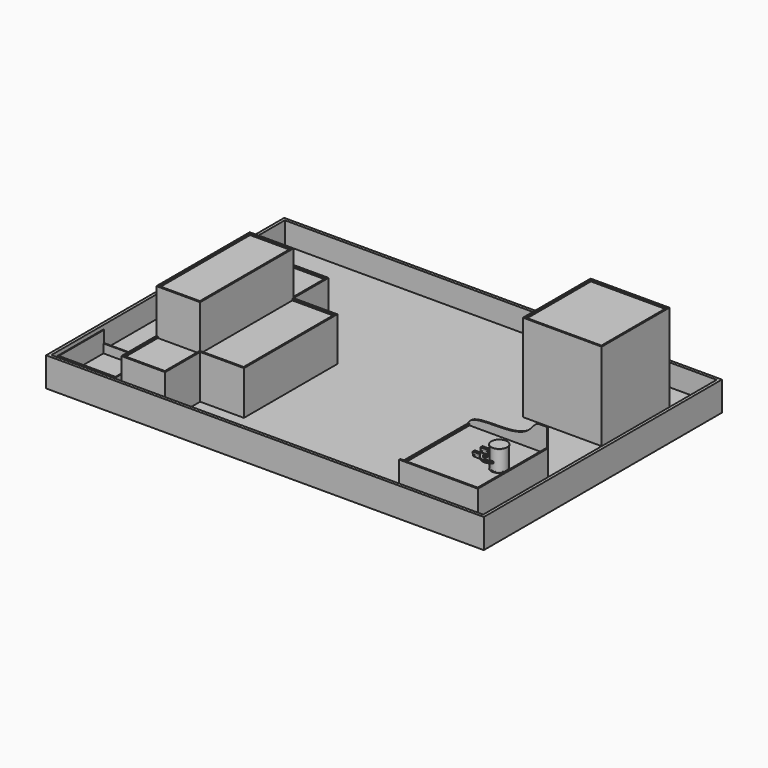
from build123d import *

# Parameters (mm, degrees)
F0_R      = 27.2
F1_DEPTH  = 2.83
F2_R      = 26.4
F3_DEPTH  = 67.36
F4_R      = 27.2
F5_DEPTH  = 2.83
F9_W      = 270
F9_H      = 300
F10_DEPTH = 72
F12_DEPTH = 15
F14_DEPTH = 5
F15_W     = 5
F15_H     = 290
F16_DEPTH = 5
F17_W     = 1500
F17_H     = 1020
F18_DEPTH = 25
F19_W     = 270
F19_H     = 290
F20_DEPTH = 300
F21_W     = 260
F21_H     = 280
F22_DEPTH = 5
F23_W     = 1500
F23_H     = 1020
F23_W_2   = 1480
F23_H_2   = 1000
F24_DEPTH = 75
F26_DEPTH = 150
F27_W     = 150
F27_H     = 400
F28_DEPTH = 150
F29_W     = 140
F29_H     = 390
F30_DEPTH = 5
F31_W     = 140
F31_H     = 145
F31_W_2   = 145
F31_H_2   = 390
F32_DEPTH = 5
F33_R     = 3
F34_DEPTH = 4
F35_R     = 3.99999
F35_2_R   = 3.99999
F36_R     = 3
F37_DEPTH = 8
F38_R     = 3
F39_DEPTH = 8
F40_R     = 3
F40_R_2   = 2.5
F41_DEPTH = 3
F42_R     = 3
F42_R_2   = 2.5
F43_DEPTH = 3
F45_DEPTH = 270.001
F46_W     = 200
F46_H     = 200
F46_W_2   = 194
F46_H_2   = 191
F47_DEPTH = 30
F49_DEPTH = 40
F50_R     = 2.5606570607
F50_R_2   = 2.9751201613
F50_R_3   = 2.7939654693
F50_R_4   = 2.7154091921
F51_DEPTH = 6


# Not quite as in the source:
# - a fillet or chamfer is up to 0.001 mm smaller than in the source, because OpenCascade refuses the exact size
# - a feature names something its author has since deleted; it is built from what else it names


with BuildPart() as f1:
    # F0 (on Top) → F1 (new body)
    with BuildSketch(Plane.XY):
        Circle(F0_R)
    extrude(amount=F1_DEPTH)

    # F2 (on face) → F3 (join)
    with BuildSketch(Plane.XY.offset(2.83)):
        Circle(F2_R)
    extrude(amount=F3_DEPTH)

    # F4 (on face) → F5 (join)
    with BuildSketch(Plane.XY.offset(70.19)):
        Circle(F4_R)
    extrude(amount=F5_DEPTH)


with BuildPart() as f10:
    # F9 (on Top) → F10 (new body)
    with BuildSketch(Plane.XY):
        with Locations((-87.8, 0)):
            Rectangle(F9_W, F9_H)
    extrude(amount=-F10_DEPTH)

    # F11 (on face) → F12 (join)
    with BuildSketch(Plane.XY):
        Polygon((-222.8, -145), (-222.8, -150), (47.2, -150), (47.2, 150), (42.2, 150), (42.2, -145), align=None)
    extrude(amount=F12_DEPTH)

    # F13 (on face) → F14 (join)
    with BuildSketch(Plane(origin=(0, 150, 0), x_dir=(-1, 0, 0), z_dir=(0, 1, 0))):
        with BuildLine():
            Line((-21.3134280931, 81.3575685024), (-47.2, 81.3575685024))
            Line((-47.2, 81.3575685024), (-47.2, -72))
            Line((-47.2, -72), (222.8, -72))
            Line((222.8, -72), (222.8, 0))
            add(Edge.make_bspline(
                [(-21.3134280931, 81.3575685024), (-6.3059147253, 81.3822787863), (12.9585432644, 38.1268753575), (103.6097013063, 23.6068887567), (223.0224295336, 30.7718731823), (222.8, 0)],
                knots=[0, 0, 0, 0, 0.2487100673, 0.6151112321, 1, 1, 1, 1], degree=3))
        make_face()
    extrude(amount=-F14_DEPTH)

    # F15 (on face) → F16 (join)
    with BuildSketch(Plane.XY):
        with Locations((-220.3, 0)):
            Rectangle(F15_W, F15_H)
    extrude(amount=F16_DEPTH)

    # F17 (on face) → F18 (join)
    with BuildSketch(Plane(origin=(0, 0, -72), x_dir=(1, 0, 0), z_dir=(0, 0, -1))):
        with Locations((-602.8, -260)):
            Rectangle(F17_W, F17_H)
    extrude(amount=F18_DEPTH)

    # F19 (on face) → F20 (join)
    with BuildSketch(Plane.XY.offset(-72)):
        with Locations((-87.8, 525)):
            Rectangle(F19_W, F19_H)
    extrude(amount=F20_DEPTH)

    # F21 (on face) → F22 (cut)
    with BuildSketch(Plane.XY.offset(228)):
        with Locations((-87.8, 525)):
            Rectangle(F21_W, F21_H)
    extrude(amount=-F22_DEPTH, mode=Mode.SUBTRACT)

    # F23 (on face) → F24 (join)
    with BuildSketch(Plane.XY.offset(-72)):
        with Locations((-602.8, 260)):
            Rectangle(F23_W, F23_H)
        with Locations((-602.8, 260)):
            Rectangle(F23_W_2, F23_H_2, mode=Mode.SUBTRACT)
    extrude(amount=F24_DEPTH)

    # F25 (on face) → F26 (join)
    with BuildSketch(Plane.XY.offset(-72)):
        Polygon((-952.8, 460), (-1102.8, 460), (-1102.8, -240), (-952.8, -240), (-952.8, -90), (-802.8, -90), (-802.8, 310), (-952.8, 310), align=None)
    extrude(amount=F26_DEPTH)

    # F27 (on face) → F28 (join)
    with BuildSketch(Plane.XY.offset(78)):
        with Locations((-1027.8, 110)):
            Rectangle(F27_W, F27_H)
    extrude(amount=F28_DEPTH)

    # F29 (on face) → F30 (cut)
    with BuildSketch(Plane.XY.offset(228)):
        with Locations((-1027.8, 110)):
            Rectangle(F29_W, F29_H)
    extrude(amount=-F30_DEPTH, mode=Mode.SUBTRACT)

    # F31 (on face) → F32 (cut)
    with BuildSketch(Plane.XY.offset(78)):
        with Locations((-1027.8, 382.5)):
            Rectangle(F31_W, F31_H)
        with Locations((-880.3, 110)):
            Rectangle(F31_W_2, F31_H_2)
        with Locations((-1027.8, -162.5)):
            Rectangle(F31_W, F31_H)
    extrude(amount=-F32_DEPTH, mode=Mode.SUBTRACT)

    # F46 (on face) → F47 (join)
    with BuildSketch(Plane.XY.offset(-72)):
        with Locations((-1232.8, -130)):
            Rectangle(F46_W, F46_H)
        with Locations((-1232.8, -128.5)):
            Rectangle(F46_W_2, F46_H_2, mode=Mode.SUBTRACT)
    extrude(amount=F47_DEPTH)

    # F48 (on face) → F49 (join)
    with BuildSketch(Plane.XY.offset(-42)):
        Polygon((-1329.8, -30), (-1332.8, -30), (-1332.8, -230), (-1329.8, -230), (-1135.8, -230), (-1132.8, -230), (-1132.8, -30), (-1135.8, -30), (-1135.8, -224), (-1329.8, -224), align=None)
    extrude(amount=F49_DEPTH)


with BuildPart() as f34:
    # F33 (on offset) → F34 (new body, symmetric)
    with BuildSketch(Plane.XY.offset(25)):
        with BuildLine():
            Line((-55, -12), (-74.5, -12))
            Line((-74.5, -12), (-74.5, -13))
            Line((-74.5, -13), (-65.6457513111, -13))
            ThreePointArc((-65.6457513111, -13), (-67, -16), (-65.6457513111, -19))
            Line((-65.6457513111, -19), (-74.5, -19))
            Line((-74.5, -19), (-74.5, -20))
            Line((-74.5, -20), (-55, -20))
            ThreePointArc((-55, -20), (-51, -16), (-55, -12))
        make_face()
        with Locations((-63, -16)):
            Circle(F33_R, mode=Mode.SUBTRACT)
        with Locations((-55, -16)):
            Circle(F33_R, mode=Mode.SUBTRACT)
    extrude(amount=F34_DEPTH, both=True)

    # F35 (radius 4 in the source; OpenCascade refuses exactly that, so slightly less here)
    f35_edges = [f34.edges().sort_by_distance(p)[0] for p in [
        (-74.5, -19.5, 29),
        (-74.5, -12.5, 29),
        (-74.5, -19.5, 21),
        (-74.5, -12.5, 21),
    ]]
    fillet(f35_edges, radius=F35_R)

    # F36 (on face) → F37 (join, through all)
    with BuildSketch(Plane.XZ.offset(20)):
        with Locations((-70.5, 25)):
            Circle(F36_R)
    extrude(amount=-F37_DEPTH)

    # F42 (on offset) → F43 (join, symmetric)
    with BuildSketch(Plane.XY.offset(25)):
        with Locations((-63, -16)):
            Circle(F42_R)
        with Locations((-63, -16)):
            Circle(F42_R_2, mode=Mode.SUBTRACT)
        with Locations((-55, -16)):
            Circle(F42_R)
        with Locations((-55, -16)):
            Circle(F42_R_2, mode=Mode.SUBTRACT)
    extrude(amount=F43_DEPTH, both=True)


with BuildPart() as f34b:
    # F33 (on offset) → F34, piece 2 (new body, symmetric)
    with BuildSketch(Plane.XY.offset(25)):
        with BuildLine():
            Line((-74.5, 13), (-74.5, 12))
            Line((-74.5, 12), (-55, 12))
            ThreePointArc((-55, 12), (-51, 16), (-55, 20))
            Line((-55, 20), (-74.5, 20))
            Line((-74.5, 20), (-74.5, 19))
            Line((-74.5, 19), (-65.6457513111, 19))
            ThreePointArc((-65.6457513111, 19), (-67, 16), (-65.6457513111, 13))
            Line((-65.6457513111, 13), (-74.5, 13))
        make_face()
        with Locations((-63, 16)):
            Circle(F33_R, mode=Mode.SUBTRACT)
        with Locations((-55, 16)):
            Circle(F33_R, mode=Mode.SUBTRACT)
    extrude(amount=F34_DEPTH, both=True)

    # F35#2 (radius 4 in the source; OpenCascade refuses exactly that, so slightly less here)
    f35_2_edges = [f34b.edges().sort_by_distance(p)[0] for p in [
        (-74.5, 12.5, 29),
        (-74.5, 19.5, 29),
        (-74.5, 19.5, 21),
        (-74.5, 12.5, 21),
    ]]
    fillet(f35_2_edges, radius=F35_2_R)

    # F38 (on face) → F39 (join, through all)
    with BuildSketch(Plane(origin=(0, 20, 0), x_dir=(-1, 0, 0), z_dir=(0, 1, 0))):
        with Locations((70.5, 25)):
            Circle(F38_R)
    extrude(amount=-F39_DEPTH)

    # F40 (on offset) → F41 (join, symmetric)
    with BuildSketch(Plane.XY.offset(25)):
        with Locations((-55, 16)):
            Circle(F40_R)
        with Locations((-55, 16)):
            Circle(F40_R_2, mode=Mode.SUBTRACT)
        with Locations((-63, 16)):
            Circle(F40_R)
        with Locations((-63, 16)):
            Circle(F40_R_2, mode=Mode.SUBTRACT)
    extrude(amount=F41_DEPTH, both=True)


with BuildPart() as f45_tool:
    # F44 (on face) → F45 (new body, through all)
    with BuildSketch(Plane(origin=(0, 20, 0), x_dir=(-1, 0, 0), z_dir=(0, 1, 0))):
        with BuildLine():
            Line((71.5, 26), (71.5, 27.2912878475))
            ThreePointArc((71.5, 27.2912878475), (70.5, 27.5), (69.5, 27.2912878475))
            Line((69.5, 27.2912878475), (69.5, 26))
            Line((69.5, 26), (68.2087121525, 26))
            ThreePointArc((68.2087121525, 26), (68, 25), (68.2087121525, 24))
            Line((68.2087121525, 24), (69.5, 24))
            Line((69.5, 24), (69.5, 22.7087121525))
            ThreePointArc((69.5, 22.7087121525), (70.5, 22.5), (71.5, 22.7087121525))
            Line((71.5, 22.7087121525), (71.5, 24))
            Line((71.5, 24), (72.7912878475, 24))
            ThreePointArc((72.7912878475, 24), (73, 25), (72.7912878475, 26))
            Line((72.7912878475, 26), (71.5, 26))
        make_face()
    extrude(amount=-F45_DEPTH)


with BuildPart() as f34_1:
    add(f34.part)

    # F45: cut by f45_tool
    add(f45_tool.part, mode=Mode.SUBTRACT)


with BuildPart() as f34b_1:
    add(f34b.part)

    # F45: cut by f45_tool
    add(f45_tool.part, mode=Mode.SUBTRACT)


with BuildPart() as f51:
    # F50 (on face) → F51 (new body)
    with BuildSketch(Plane.XY.offset(29)):
        with BuildLine():
            ThreePointArc((-2.4018440386, -30.2), (-23.8352456668, -33.5517809086), (-39.8274711859, -18.8932044578))
            Line((-39.8274711859, -18.8932044578), (-29.2851294938, -15.0561058824))
            ThreePointArc((-29.2851294938, -15.0561058824), (-32.2874871641, -1.6301629169), (-29.2851294938, 11.7957800485))
            Line((-29.2851294938, 11.7957800485), (-39.8274711859, 15.6328786239))
            ThreePointArc((-39.8274711859, 15.6328786239), (-24.780937365, 32.335789608), (-2.4018440386, 30.2))
            Line((-2.4018440386, 30.2), (3.890708183, 30.2))
            ThreePointArc((3.890708183, 30.2), (-23.9645202209, 39.6314204929), (-46.4946061887, 20.7300801112))
            Line((-46.4946061887, 20.7300801112), (-73.7728578303, 20.7300801112))
            Line((-73.7728578303, 20.7300801112), (-73.8147060448, 11.7957800485))
            Line((-73.8147060448, 11.7957800485), (-46.4946061887, 11.7957800485))
            Line((-46.4946061887, 11.7957800485), (-35.2182947393, 7.6915383286))
            ThreePointArc((-35.2182947393, 7.6915383286), (-37.636454775, -0.766008443), (-35.2182947393, -9.2235552147))
            Line((-35.2182947393, -9.2235552147), (-46.4946061887, -11.3503415921))
            Line((-46.4946061887, -11.3503415921), (-74.5422616601, -11.3503415921))
            Line((-74.5422616601, -11.3503415921), (-74.5422616601, -20.5755829811))
            Line((-74.5422616601, -20.5755829811), (-47.0614409433, -20.5755829811))
            ThreePointArc((-47.0614409433, -20.5755829811), (-24.4330972816, -40.4638225143), (3.890708183, -30.2))
            Line((3.890708183, -30.2), (-2.4018440386, -30.2))
        make_face()
        with Locations((-63, -16)):
            Circle(F50_R, mode=Mode.SUBTRACT)
        with Locations((-55, -16.1286499351)):
            Circle(F50_R_2, mode=Mode.SUBTRACT)
        with Locations((-63, 16)):
            Circle(F50_R_3, mode=Mode.SUBTRACT)
        with Locations((-55, 16)):
            Circle(F50_R_4, mode=Mode.SUBTRACT)
    extrude(amount=F51_DEPTH)


solid = Compound([f1.part, f10.part, f34_1.part, f34b_1.part, f51.part])
